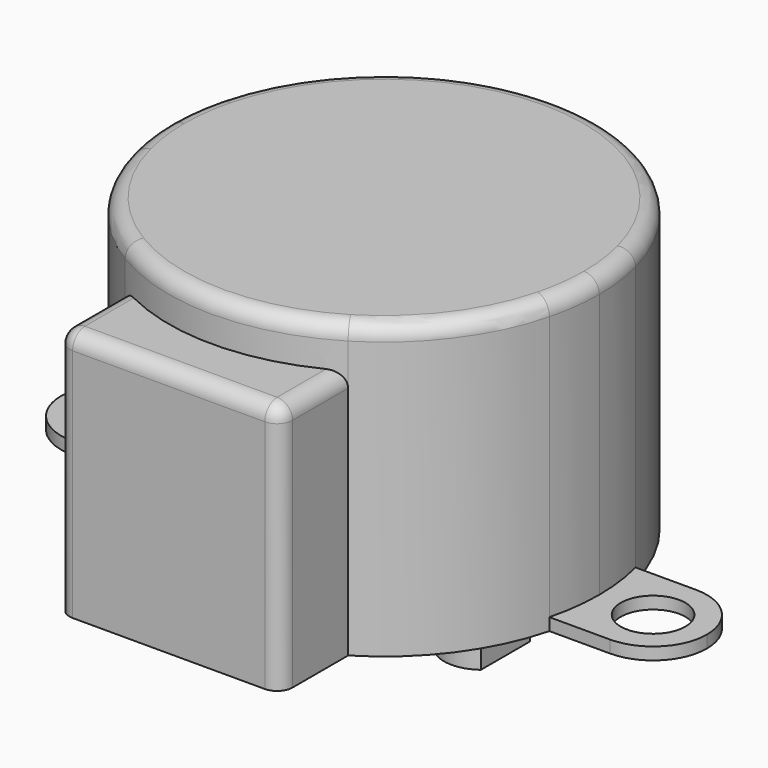
from build123d import *

# Parameters (mm, degrees)
F0_R     = 4.5
F1_DEPTH = 19
F2_DEPTH = 10
F3_DEPTH = 1.5
F0_R_2   = 2.1
F4_DEPTH = 0.8
F5_DEPTH = 16.3
F6_R     = 1
F7_DEPTH = 4


with BuildPart() as f1:
    # F0 (on Top) → F1 (new body)
    with BuildSketch(Plane.XY):
        with BuildLine():
            ThreePointArc((13.5554417117, -3.5), (13.8884157477, -1.7640600948), (14, 0))
            ThreePointArc((14, 0), (13.8884157477, 1.7640600948), (13.5554417117, 3.5))
            ThreePointArc((13.5554417117, 3.5), (0, 14), (-13.5554417117, 3.5))
            ThreePointArc((-13.5554417117, 3.5), (-13.8884157477, 1.7640600948), (-14, 0))
            ThreePointArc((-14, 0), (-13.8884157477, -1.7640600948), (-13.5554417117, -3.5))
            ThreePointArc((-13.5554417117, -3.5), (-11.2329663029, -8.3558642903), (-7.25, -11.976539567))
            ThreePointArc((-7.25, -11.976539567), (0, -14), (7.25, -11.976539567))
            ThreePointArc((7.25, -11.976539567), (11.2329663029, -8.3558642903), (13.5554417117, -3.5))
        make_face()
        with Locations((0, 8)):
            Circle(F0_R, mode=Mode.SUBTRACT)
        with Locations((0, 8)):
            Circle(F0_R)
        with BuildLine():
            ThreePointArc((1.5, 10), (2.2360679775, 9.1180339887), (2.5, 8))
            ThreePointArc((2.5, 8), (2.2360679775, 6.8819660113), (1.5, 6))
            ThreePointArc((1.5, 6), (0, 5.5), (-1.5, 6))
            ThreePointArc((-1.5, 6), (-2.5, 8), (-1.5, 10))
            ThreePointArc((-1.5, 10), (0, 10.5), (1.5, 10))
        make_face(mode=Mode.SUBTRACT)
        with BuildLine():
            Line((1.5, 6), (1.5, 10))
            ThreePointArc((1.5, 10), (0, 10.5), (-1.5, 10))
            Line((-1.5, 10), (-1.5, 6))
            ThreePointArc((-1.5, 6), (0, 5.5), (1.5, 6))
        make_face()
        with BuildLine():
            ThreePointArc((1.5, 6), (2.2360679775, 6.8819660113), (2.5, 8))
            ThreePointArc((2.5, 8), (2.2360679775, 9.1180339887), (1.5, 10))
            Line((1.5, 10), (1.5, 6))
        make_face()
        with BuildLine():
            Line((-1.5, 6), (-1.5, 10))
            ThreePointArc((-1.5, 10), (-2.5, 8), (-1.5, 6))
        make_face()
    extrude(amount=F1_DEPTH)

    # F0 (on Top) → F3 (join)
    with BuildSketch(Plane.XY):
        with Locations((0, 8)):
            Circle(F0_R)
        with BuildLine():
            ThreePointArc((1.5, 10), (2.2360679775, 9.1180339887), (2.5, 8))
            ThreePointArc((2.5, 8), (2.2360679775, 6.8819660113), (1.5, 6))
            ThreePointArc((1.5, 6), (0, 5.5), (-1.5, 6))
            ThreePointArc((-1.5, 6), (-2.5, 8), (-1.5, 10))
            ThreePointArc((-1.5, 10), (0, 10.5), (1.5, 10))
        make_face(mode=Mode.SUBTRACT)
    extrude(amount=-F3_DEPTH)

    # F0 (on Top) → F4 (join)
    with BuildSketch(Plane.XY):
        with BuildLine():
            ThreePointArc((17.5, -3.5), (15.0251262658, -2.4748737342), (14, 0))
            ThreePointArc((14, 0), (13.8884157477, -1.7640600948), (13.5554417117, -3.5))
            Line((13.5554417117, -3.5), (17.5, -3.5))
        make_face()
        with BuildLine():
            ThreePointArc((17.5, 3.5), (15.0251262658, 2.4748737342), (14, 0))
            ThreePointArc((14, 0), (15.0251262658, -2.4748737342), (17.5, -3.5))
            ThreePointArc((17.5, -3.5), (19.9748737342, -2.4748737342), (21, 0))
            ThreePointArc((21, 0), (19.9748737342, 2.4748737342), (17.5, 3.5))
        make_face()
        with Locations((17.5, 0)):
            Circle(F0_R_2, mode=Mode.SUBTRACT)
        with BuildLine():
            ThreePointArc((13.5554417117, 3.5), (13.8884157477, 1.7640600948), (14, 0))
            ThreePointArc((14, 0), (15.0251262658, 2.4748737342), (17.5, 3.5))
            Line((17.5, 3.5), (13.5554417117, 3.5))
        make_face()
        with BuildLine():
            ThreePointArc((-13.5554417117, -3.5), (-13.8884157477, -1.7640600948), (-14, 0))
            ThreePointArc((-14, 0), (-15.0251262658, -2.4748737342), (-17.5, -3.5))
            Line((-17.5, -3.5), (-13.5554417117, -3.5))
        make_face()
        with BuildLine():
            ThreePointArc((-17.5, -3.5), (-15.0251262658, -2.4748737342), (-14, 0))
            ThreePointArc((-14, 0), (-15.0251262658, 2.4748737342), (-17.5, 3.5))
            ThreePointArc((-17.5, 3.5), (-21, 0), (-17.5, -3.5))
        make_face()
        with Locations((-17.5, 0)):
            Circle(F0_R_2, mode=Mode.SUBTRACT)
        with BuildLine():
            ThreePointArc((-14, 0), (-13.8884157477, 1.7640600948), (-13.5554417117, 3.5))
            Line((-13.5554417117, 3.5), (-17.5, 3.5))
            ThreePointArc((-17.5, 3.5), (-15.0251262658, 2.4748737342), (-14, 0))
        make_face()
    extrude(amount=F4_DEPTH)

    # F0 (on Top) → F5 (join, through all)
    with BuildSketch(Plane.XY):
        with BuildLine():
            Line((7.25, -17.5), (7.25, -11.976539567))
            ThreePointArc((7.25, -11.976539567), (0, -14), (-7.25, -11.976539567))
            Line((-7.25, -11.976539567), (-7.25, -17.5))
            Line((-7.25, -17.5), (7.25, -17.5))
        make_face()
    extrude(amount=F5_DEPTH)

    # F6
    f6_edges = [f1.edges().sort_by_distance(p)[0] for p in [
        (-13.555442, 3.5, 19),
        (-7.25, -17.5, 8.15),
        (7.25, -17.5, 8.15),
        (0, -17.5, 16.3),
        (-7.25, -14.73827, 16.3),
        (7.25, -14.73827, 16.3),
    ]]
    fillet(f6_edges, radius=F6_R)


with BuildPart() as f2:
    # F0 (on Top) → F2 (new body)
    with BuildSketch(Plane.XY):
        with BuildLine():
            Line((1.5, 6), (1.5, 10))
            ThreePointArc((1.5, 10), (0, 10.5), (-1.5, 10))
            Line((-1.5, 10), (-1.5, 6))
            ThreePointArc((-1.5, 6), (0, 5.5), (1.5, 6))
        make_face()
    extrude(amount=-F2_DEPTH)

    # F0 (on Top) → F7 (join)
    with BuildSketch(Plane.XY):
        with BuildLine():
            Line((-1.5, 6), (-1.5, 10))
            ThreePointArc((-1.5, 10), (-2.5, 8), (-1.5, 6))
        make_face()
        with BuildLine():
            ThreePointArc((1.5, 6), (2.2360679775, 6.8819660113), (2.5, 8))
            ThreePointArc((2.5, 8), (2.2360679775, 9.1180339887), (1.5, 10))
            Line((1.5, 10), (1.5, 6))
        make_face()
    extrude(amount=-F7_DEPTH)


solid = Compound([f1.part, f2.part])
